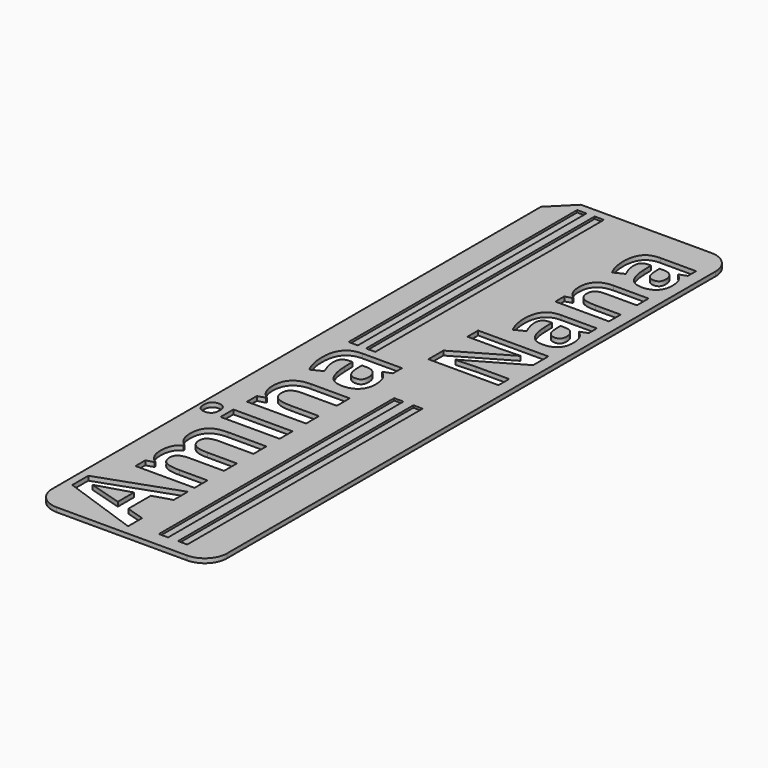
from build123d import *

# Parameters (mm, degrees)
F0_W           = 40
F0_H           = 150
F1_DEPTH       = 1
F2_TEXT_SIZE   = 24.7845870849
F2_TEXT_SIZE_2 = 22.4903361837
F3_DEPTH       = 25.4
F4_SIZE        = 5.08
F5_R           = 5.08
F6_W           = 2.1168552339
F6_H           = 67.3544239253
F6_H_2         = 65.4184622507
F7_DEPTH       = 0.5


# Not quite as in the source:
# - Text() gives the source's letters only with a copy of the font that has no kerning and outlines rounded to 1/6400 em; it was checked with that copy


with BuildPart() as f1:
    # F0 (on Top) → F1 (new body)
    with BuildSketch(Plane.XY):
        Rectangle(F0_W, F0_H)
    extrude(amount=F1_DEPTH)

    # F2 (on face) → F3 (cut)
    with BuildSketch(Plane.XY.offset(1)):
        with Locations(Location((-0.3770940235, -72.7660059929), (0, 0, 90))):
            Text('Amina', F2_TEXT_SIZE, font='Open Sans', font_style=FontStyle.BOLD, text_align=(TextAlign.LEFT, TextAlign.BOTTOM))
        with Locations(Location((17.2090421052, 9.2379947007), (0, 0, 90))):
            Text('Nana', F2_TEXT_SIZE_2, font='Open Sans', font_style=FontStyle.BOLD, text_align=(TextAlign.LEFT, TextAlign.BOTTOM))
    extrude(amount=-F3_DEPTH, mode=Mode.SUBTRACT)

    # F4
    f4_edges = [f1.edges().sort_by_distance(p)[0] for p in [
        (-20, 75, 0.5),
    ]]
    chamfer(f4_edges, length=F4_SIZE)

    # F5
    f5_edges = [f1.edges().sort_by_distance(p)[0] for p in [
        (-20, -75, 0.5),
        (20, -75, 0.5),
        (20, 75, 0.5),
    ]]
    fillet(f5_edges, radius=F5_R)

    # F6 (on face) → F7 (cut)
    with BuildSketch(Plane.XY.offset(1)):
        with Locations((6.8524312228, -37.991293706)):
            Rectangle(F6_W, F6_H)
        with Locations((11.2439803779, -37.991293706)):
            Rectangle(F6_W, F6_H)
        with Locations((-13.1012201309, 40.2720612382)):
            Rectangle(F6_W, F6_H_2)
        with Locations((-9.1085783051, 40.2720612382)):
            Rectangle(F6_W, F6_H_2)
    extrude(amount=-F7_DEPTH, mode=Mode.SUBTRACT)


solid = f1.part
